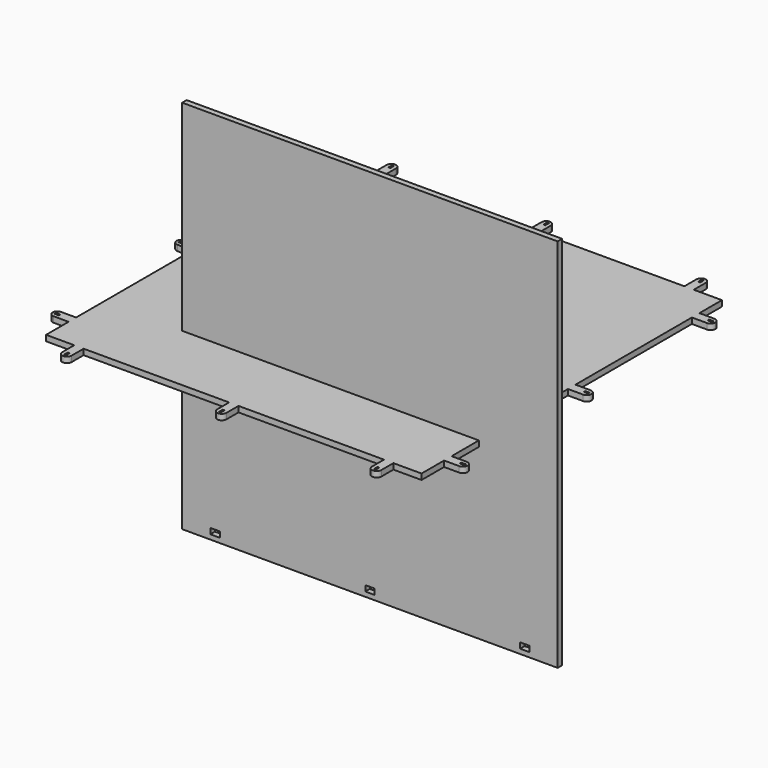
from build123d import *

# Parameters (mm, degrees)
F0_W     = 5
F0_H     = 2
F0_W_2   = 2
F0_H_2   = 5
F1_DEPTH = 6.1
F2_W     = 400
F2_H     = 400
F2_W_2   = 10
F2_H_2   = 6
F3_DEPTH = 6


# Not quite as in the source:
# - a feature names something its author has since deleted; it is built from what else it names


with BuildPart() as f1:
    # F0 (on Top) → F1 (new body)
    with BuildSketch(Plane.XY):
        Polygon((-263.8466370106, 317.6659622788), (-293.8466370106, 317.6659622788), (-293.8466370106, 287.6659622788), (-293.8466370106, 277.6659622788), (-293.8466370106, 122.6659622788), (-293.8466370106, 112.6659622788), (-293.8466370106, -42.3340377212), (-293.8466370106, -52.3340377212), (-293.8466370106, -82.3340377212), (-263.8466370106, -82.3340377212), (-253.8466370106, -82.3340377212), (-98.8466370106, -82.3340377212), (-88.8466370106, -82.3340377212), (66.1533629894, -82.3340377212), (76.1533629894, -82.3340377212), (106.1533629894, -82.3340377212), (106.1533629894, -52.3340377212), (106.1533629894, -42.3340377212), (106.1533629894, 112.6659622788), (106.1533629894, 122.6659622788), (106.1533629894, 277.6659622788), (106.1533629894, 287.6659622788), (106.1533629894, 317.6659622788), (76.1533629894, 317.6659622788), (66.1533629894, 317.6659622788), (-88.8466370106, 317.6659622788), (-98.8466370106, 317.6659622788), (-253.8466370106, 317.6659622788), align=None)
        with BuildLine():
            Line((-293.8466370106, -52.3340377212), (-293.8466370106, -42.3340377212))
            Line((-293.8466370106, -42.3340377212), (-309.8466370106, -42.3340377212))
            ThreePointArc((-309.8466370106, -42.3340377212), (-314.8466370106, -47.3340377212), (-309.8466370106, -52.3340377212))
            Line((-309.8466370106, -52.3340377212), (-293.8466370106, -52.3340377212))
        make_face()
        with Locations((-309.8466370106, -47.3340377212)):
            Rectangle(F0_W, F0_H, mode=Mode.SUBTRACT)
        with BuildLine():
            Line((-293.8466370106, 112.6659622788), (-293.8466370106, 122.6659622788))
            Line((-293.8466370106, 122.6659622788), (-309.8466370106, 122.6659622788))
            ThreePointArc((-309.8466370106, 122.6659622788), (-314.8466370106, 117.6659622788), (-309.8466370106, 112.6659622788))
            Line((-309.8466370106, 112.6659622788), (-293.8466370106, 112.6659622788))
        make_face()
        with Locations((-309.8466370106, 117.6659622788)):
            Rectangle(F0_W, F0_H, mode=Mode.SUBTRACT)
        with BuildLine():
            Line((-293.8466370106, 277.6659622788), (-293.8466370106, 287.6659622788))
            Line((-293.8466370106, 287.6659622788), (-309.8466370106, 287.6659622788))
            ThreePointArc((-309.8466370106, 287.6659622788), (-314.8466370106, 282.6659622788), (-309.8466370106, 277.6659622788))
            Line((-309.8466370106, 277.6659622788), (-293.8466370106, 277.6659622788))
        make_face()
        with Locations((-309.8466370106, 282.6659622788)):
            Rectangle(F0_W, F0_H, mode=Mode.SUBTRACT)
        with BuildLine():
            Line((122.1533629894, -42.3340377212), (106.1533629894, -42.3340377212))
            Line((106.1533629894, -42.3340377212), (106.1533629894, -52.3340377212))
            Line((106.1533629894, -52.3340377212), (122.1533629894, -52.3340377212))
            ThreePointArc((122.1533629894, -52.3340377212), (127.1533629894, -47.3340377212), (122.1533629894, -42.3340377212))
        make_face()
        with Locations((122.1533629894, -47.3340377212)):
            Rectangle(F0_W, F0_H, mode=Mode.SUBTRACT)
        with BuildLine():
            Line((122.1533629894, 122.6659622788), (106.1533629894, 122.6659622788))
            Line((106.1533629894, 122.6659622788), (106.1533629894, 112.6659622788))
            Line((106.1533629894, 112.6659622788), (122.1533629894, 112.6659622788))
            ThreePointArc((122.1533629894, 112.6659622788), (127.1533629894, 117.6659622788), (122.1533629894, 122.6659622788))
        make_face()
        with Locations((122.1533629894, 117.6659622788)):
            Rectangle(F0_W, F0_H, mode=Mode.SUBTRACT)
        with BuildLine():
            Line((122.1533629894, 287.6659622788), (106.1533629894, 287.6659622788))
            Line((106.1533629894, 287.6659622788), (106.1533629894, 277.6659622788))
            Line((106.1533629894, 277.6659622788), (122.1533629894, 277.6659622788))
            ThreePointArc((122.1533629894, 277.6659622788), (127.1533629894, 282.6659622788), (122.1533629894, 287.6659622788))
        make_face()
        with Locations((122.1533629894, 282.6659622788)):
            Rectangle(F0_W, F0_H, mode=Mode.SUBTRACT)
        with BuildLine():
            Line((-253.8466370106, -82.3340377212), (-263.8466370106, -82.3340377212))
            Line((-263.8466370106, -82.3340377212), (-263.8466370106, -98.3340377212))
            ThreePointArc((-263.8466370106, -98.3340377212), (-258.8466370106, -103.3340377212), (-253.8466370106, -98.3340377212))
            Line((-253.8466370106, -98.3340377212), (-253.8466370106, -82.3340377212))
        make_face()
        with Locations((-258.8466370106, -98.3340377212)):
            Rectangle(F0_W_2, F0_H_2, mode=Mode.SUBTRACT)
        with BuildLine():
            Line((-88.8466370106, -82.3340377212), (-98.8466370106, -82.3340377212))
            Line((-98.8466370106, -82.3340377212), (-98.8466370106, -98.3340377212))
            ThreePointArc((-98.8466370106, -98.3340377212), (-93.8466370106, -103.3340377212), (-88.8466370106, -98.3340377212))
            Line((-88.8466370106, -98.3340377212), (-88.8466370106, -82.3340377212))
        make_face()
        with Locations((-93.8466370106, -98.3340377212)):
            Rectangle(F0_W_2, F0_H_2, mode=Mode.SUBTRACT)
        with BuildLine():
            Line((76.1533629894, -82.3340377212), (66.1533629894, -82.3340377212))
            Line((66.1533629894, -82.3340377212), (66.1533629894, -98.3340377212))
            ThreePointArc((66.1533629894, -98.3340377212), (71.1533629894, -103.3340377212), (76.1533629894, -98.3340377212))
            Line((76.1533629894, -98.3340377212), (76.1533629894, -82.3340377212))
        make_face()
        with Locations((71.1533629894, -98.3340377212)):
            Rectangle(F0_W_2, F0_H_2, mode=Mode.SUBTRACT)
        with BuildLine():
            Line((66.1533629894, 333.6659622788), (66.1533629894, 317.6659622788))
            Line((66.1533629894, 317.6659622788), (76.1533629894, 317.6659622788))
            Line((76.1533629894, 317.6659622788), (76.1533629894, 333.6659622788))
            ThreePointArc((76.1533629894, 333.6659622788), (71.1533629894, 338.6659622788), (66.1533629894, 333.6659622788))
        make_face()
        with Locations((71.1533629894, 333.6659622788)):
            Rectangle(F0_W_2, F0_H_2, mode=Mode.SUBTRACT)
        with BuildLine():
            Line((-98.8466370106, 333.6659622788), (-98.8466370106, 317.6659622788))
            Line((-98.8466370106, 317.6659622788), (-88.8466370106, 317.6659622788))
            Line((-88.8466370106, 317.6659622788), (-88.8466370106, 333.6659622788))
            ThreePointArc((-88.8466370106, 333.6659622788), (-93.8466370106, 338.6659622788), (-98.8466370106, 333.6659622788))
        make_face()
        with Locations((-93.8466370106, 333.6659622788)):
            Rectangle(F0_W_2, F0_H_2, mode=Mode.SUBTRACT)
        with BuildLine():
            Line((-263.8466370106, 333.6659622788), (-263.8466370106, 317.6659622788))
            Line((-263.8466370106, 317.6659622788), (-253.8466370106, 317.6659622788))
            Line((-253.8466370106, 317.6659622788), (-253.8466370106, 333.6659622788))
            ThreePointArc((-253.8466370106, 333.6659622788), (-258.8466370106, 338.6659622788), (-263.8466370106, 333.6659622788))
        make_face()
        with Locations((-258.8466370106, 333.6659622788)):
            Rectangle(F0_W_2, F0_H_2, mode=Mode.SUBTRACT)
    extrude(amount=-F1_DEPTH)


with BuildPart() as f3:
    # F2 (on Front) → F3 (new body)
    with BuildSketch(Plane.XZ):
        with Locations((-9.8858773708, 13.9629530753)):
            Rectangle(F2_W, F2_H)
        with Locations((-174.8858773708, -178.0370469247)):
            Rectangle(F2_W_2, F2_H_2, mode=Mode.SUBTRACT)
        with Locations((-9.8858773708, -178.0370469247)):
            Rectangle(F2_W_2, F2_H_2, mode=Mode.SUBTRACT)
        with Locations((155.1141226292, -178.0370469247)):
            Rectangle(F2_W_2, F2_H_2, mode=Mode.SUBTRACT)
    extrude(amount=F3_DEPTH)


solid = Compound([f1.part, f3.part])
